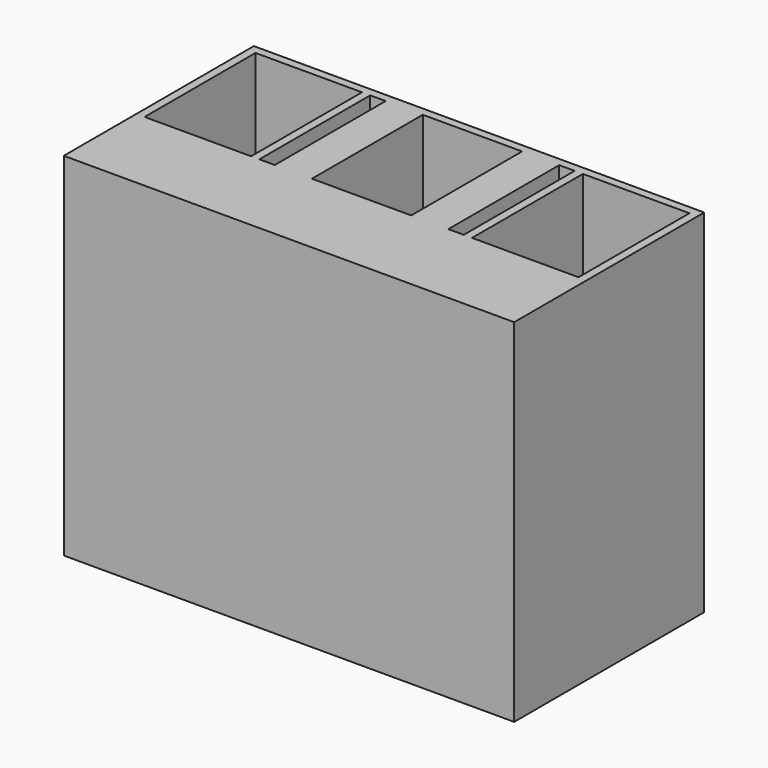
from build123d import *

# Parameters (mm, degrees)
F0_W     = 103.351444006
F0_H     = 32.4089471251
F0_R     = 8.8186134511
F2_DEPTH = 23.876
F3_T     = 2.54
F4_R     = 5.08
F5_DEPTH = 75.946
F6_DEPTH = 25.4


# Not quite as in the source:
# - a shell that OpenCascade refuses in one call is made with other operations: the cavity is built on its own and cut out
# - the program builds the solid bodies; features that only make, move or delete a surface that nothing else refers to are left out


with BuildPart() as f2:
    # F0 (on Front) → F2 (new body, symmetric)
    with BuildSketch(Plane.XZ):
        with Locations((-17.6653191447, -6.3865175471)):
            Rectangle(F0_W, F0_H)
        with Locations((-21.0040956736, 0)):
            Circle(F0_R, mode=Mode.SUBTRACT)
    extrude(amount=F2_DEPTH, both=True)

    # F3: shell of thickness 2.54, made by hand


with BuildPart() as f3_core1:
    # F3_t2: copy of F2
    add(f2.part)

    # the walls: a layer under each face that stays
    f3_faces = [f3_core1.faces().sort_by_distance(p)[0] for p in [
        (34.0104028583, 0, -6.3865175471),
        (-17.6653191447, 0, -22.5909911096),
        (-69.3410411477, 0, -6.3865175471),
        (-52.11580048, -23.876, -17.1894999221),
        (-29.8227091247, 0, 0),
        (-52.11580048, 23.876, -17.1894999221),
    ]]
    thicken(f3_faces, amount=-F3_T, mode=Mode.SUBTRACT)


with BuildPart() as f2_1:
    add(f2.part)

    # what is left inside the walls is the cavity
    f3_cavity = [f3_core1.part.solids().sort_by_distance(p)[0] for p in [
        (-17.665319, 7.112, -20.025591),
    ]]
    add(f3_cavity, mode=Mode.SUBTRACT)

    # F4
    f4_edges = [f2_1.edges().sort_by_distance(p)[0] for p in [
        (34.010403, 0, -22.590991),
    ]]
    fillet(f4_edges, radius=F4_R)

    # F5 (add): a face of the model
    f5_faces = [f2_1.faces().sort_by_distance(p)[0] for p in [
        (-18.9893309888, 0, 9.8179560155),
    ]]
    extrude(f5_faces, amount=F5_DEPTH)

    # F6 (add): a face of the model
    f6_faces = [f2_1.faces().sort_by_distance(p)[0] for p in [
        (-17.6163810634, -23.876, 32.3181446874),
    ]]
    extrude(f6_faces, amount=F6_DEPTH)

    # F7: F2 across plane


with BuildPart() as f2_2:
    add(f2_1.part)
    add(f2_1.part.mirror(Plane.YZ))


solid = f2_2.part
